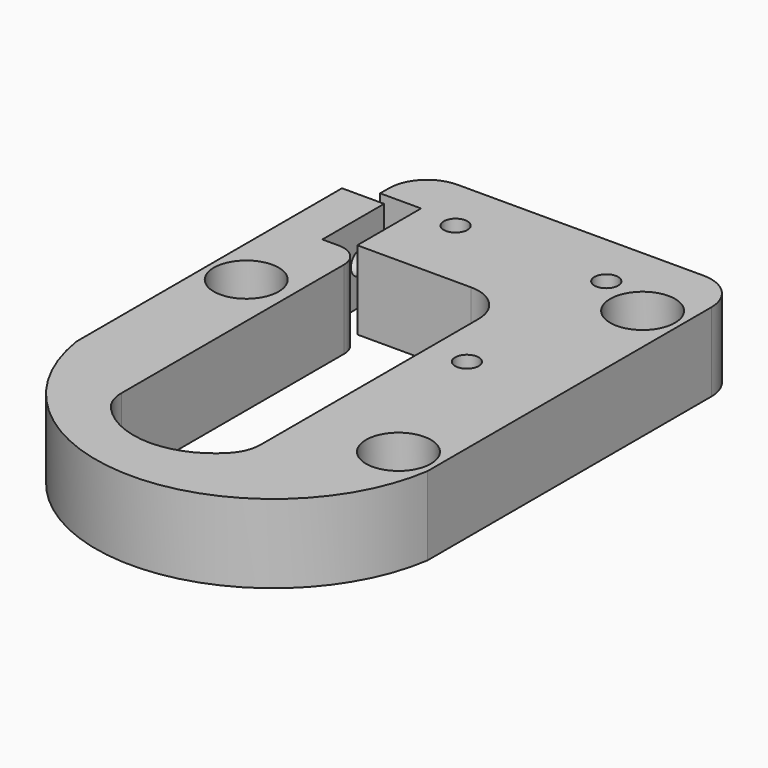
from build123d import *

# Parameters (mm, degrees)
F1_DEPTH  = 10.3
F2_R      = 1.55
F2_R_2    = 2.5
F2_W      = 18.2711938396
F2_H      = 41.0630945116
F2_W_2    = 3.7480126619
F2_H_2    = 6.4359663129
F3_DEPTH  = 10.3
F4_R      = 3
F5_R      = 5
F6_R      = 4.25
F7_DEPTH  = 5.8
F8_R      = 1.55
F9_DEPTH  = 25
F11_DEPTH = 4


with BuildPart() as f1:
    # F0 (on Top) → F1 (new body)
    with BuildSketch(Plane.XY):
        with BuildLine():
            Line((23, -15.75), (23, 35.75))
            Line((23, 35.75), (-23, 35.75))
            Line((-23, 35.75), (-23, -15.75))
            ThreePointArc((-23, -15.75), (0, -35.5223387435), (23, -15.75))
        make_face()
    extrude(amount=F1_DEPTH)

    # F2 (on face) → F3 (cut, through all)
    with BuildSketch(Plane.XY.offset(10.3)):
        with Locations((11, 28.55)):
            Circle(F2_R)
        with Locations((-8.75, 28.55)):
            Circle(F2_R)
        with Locations((11, 5.7171783878)):
            Circle(F2_R)
        with Locations((18, 25.75)):
            Circle(F2_R_2)
        with Locations((18, -14.25)):
            Circle(F2_R_2)
        with Locations((-18, 5.8170498922)):
            Circle(F2_R_2)
        with Locations((-3.1221020035, -2.9017189518)):
            Rectangle(F2_W, F2_H)
        Polygon((-12.2576989233, 17.6298283041), (6.0134949163, 17.6298283041), (6.0134949163, 18.8598968089), (-12.2576989233, 18.8598968089), (-13.8854337856, 18.8598968089), (-13.8854337856, 29.3140336871), (-15.5863631517, 29.3140336871), (-19.2519873381, 29.3140336871), (-23, 29.3140336871), (-23, 27.7502387762), (-17.4777284265, 27.7502387762), (-17.4777284265, 17.6298283041), (-15.5863631517, 17.6298283041), align=None)
        with BuildLine():
            ThreePointArc((-12.2576989233, -23.4332662076), (-3.1221020035, -28.5924931443), (6.0134949163, -23.4332662076))
            Line((6.0134949163, -23.4332662076), (-12.2576989233, -23.4332662076))
        make_face()
        with Locations((-21.125993669, 32.5320168436)):
            Rectangle(F2_W_2, F2_H_2)
    extrude(amount=-F3_DEPTH, mode=Mode.SUBTRACT)

    # F4
    f4_edges = [f1.edges().sort_by_distance(p)[0] for p in [
        (-12.257699, 17.629828, 5.15),
    ]]
    fillet(f4_edges, radius=F4_R)

    # F5
    f5_edges = [f1.edges().sort_by_distance(p)[0] for p in [
        (-19.251987, 35.75, 5.15),
        (23, 35.75, 5.15),
        (-12.257699, -23.433266, 5.15),
        (6.013495, -23.433266, 5.15),
        (6.013495, 18.859897, 5.15),
    ]]
    fillet(f5_edges, radius=F5_R)

    # F6 (on face) → F7 (cut)
    with BuildSketch(Plane.XY.offset(10.3)):
        with Locations((18, 25.75)):
            Circle(F6_R)
        with Locations((-18, 5.8170498922)):
            Circle(F6_R)
        with Locations((18, -14.25)):
            Circle(F6_R)
    extrude(amount=-F7_DEPTH, mode=Mode.SUBTRACT)

    # F8 (on face) → F9 (cut)
    with BuildSketch(Plane(origin=(-23, 0, 0), x_dir=(0, -1, 0), z_dir=(-1, 0, 0))):
        with Locations((-23.8586217165, 5.15)):
            Circle(F8_R)
    extrude(amount=-F9_DEPTH, mode=Mode.SUBTRACT)

    # F10 (on face) → F11 (cut)
    with BuildSketch(Plane(origin=(0, 0, 0), x_dir=(1, 0, 0), z_dir=(0, 0, -1))):
        Polygon((11.0856638946, -25.1447107273), (8.09376493, -26.7731682547), (8.0081010353, -30.1784575274), (10.9143361054, -31.9552892727), (13.90623507, -30.3268317453), (13.9918989647, -26.9215424726), align=None)
        Polygon((-8.7919851376, -25.1438921653), (-11.7207684817, -26.8833062784), (-11.6787833441, -30.2894141131), (-8.7080148624, -31.9561078347), (-5.7792315183, -30.2166937216), (-5.8212166559, -26.8105858869), align=None)
        Polygon((10.8521251413, -2.3140230343), (7.9788435816, -4.1436640952), (8.1267184402, -7.5468194487), (11.1478748587, -9.1203337412), (14.0211564184, -7.2906926803), (13.8732815598, -3.8875373269), align=None)
    extrude(amount=-F11_DEPTH, mode=Mode.SUBTRACT)


solid = f1.part
